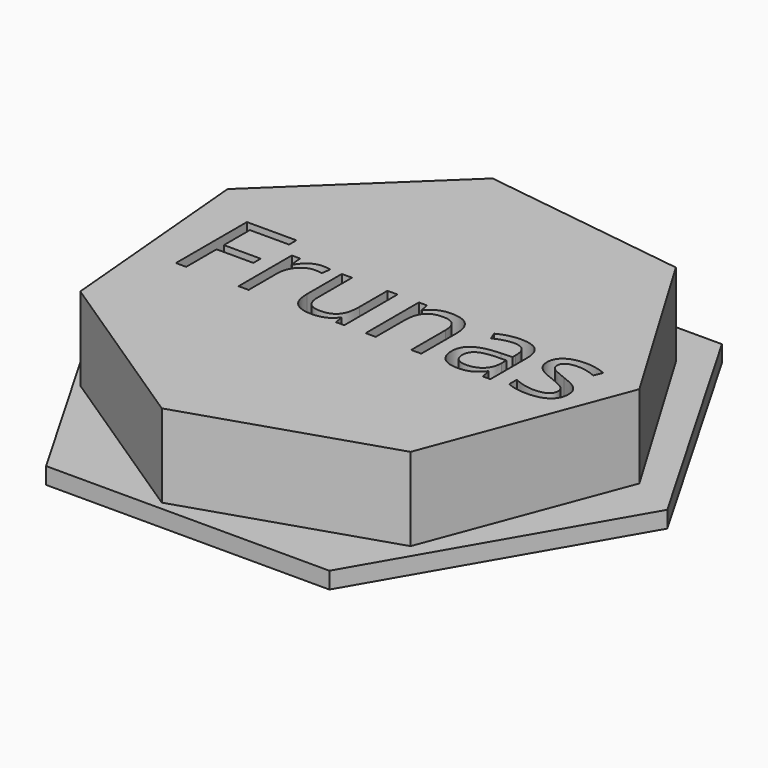
from build123d import *

# Parameters (mm, degrees)
F1_DEPTH     = 25
F2_TEXT_SIZE = 37.454279444
F3_DEPTH     = 25
F5_DEPTH     = 5


# Not quite as in the source:
# - Text() gives the source's letters only with a copy of the font that has no kerning and outlines rounded to 1/6400 em; it was checked with that copy


with BuildPart() as f1:
    # F0 (on Top) → F1 (new body)
    with BuildSketch(Plane.XY):
        Polygon((-61.9537864245, -36.8952702822), (-9.7816701614, -71.4412454425), (49.7562432429, -52.1905056488), (71.8266906429, 6.3607493907), (39.8101749913, 60.1222304034), (-22.1842144083, 68.6104456523), (-67.4734378829, 25.433595927), align=None)
    extrude(amount=F1_DEPTH)

    # F2 (on Top) → F3 (cut)
    with BuildSketch(Plane.XY):
        with Locations((-57.1019993311, -11.5703471125)):
            Text('Frunas', F2_TEXT_SIZE, font='Open Sans', text_align=(TextAlign.LEFT, TextAlign.BOTTOM))
    extrude(amount=F3_DEPTH, mode=Mode.SUBTRACT)


with BuildPart() as f5:
    # F4 (on Top) → F5 (new body)
    with BuildSketch(Plane.XY):
        Polygon((42.6624334758, 73.8935023546), (-42.6624334758, 73.8935023546), (-85.3248669516, 0), (-42.6624334758, -73.8935023546), (42.6624334758, -73.8935023546), (85.3248669516, 0), align=None)
    extrude(amount=-F5_DEPTH)


solid = Compound([f1.part, f5.part])
